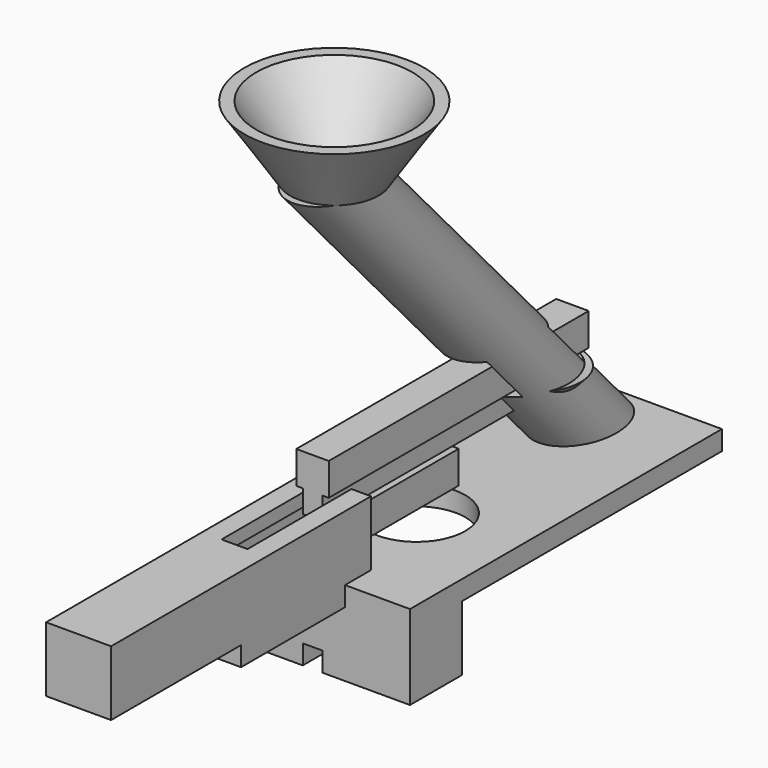
from build123d import *

# Parameters (mm, degrees)
F0_W          = 10
F0_H          = 10
F0_W_2        = 6
F0_H_2        = 6
F1_DEPTH      = 50
F2_W          = 4
F2_H          = 20
F3_DEPTH      = 3
F4_W          = 5
F4_H          = 5
F5_DEPTH      = 20
F7_DEPTH      = 25
F7_DEPTH_BACK = 25
F8_W          = 30
F8_H          = 80
F9_DEPTH      = 3
F10_R         = 7.5
F11_DEPTH     = 3.001
F12_W         = 30
F12_H         = 10
F13_DEPTH     = 10
F14_W         = 3
F14_H         = 10
F15_DEPTH     = 3
F16_R         = 1
F17_DEPTH     = 5
F18_W         = 6
F18_H         = 6
F19_DEPTH     = 2
F20_W         = 10
F20_H         = 20
F21_DEPTH     = 25
F25_W         = 7.5
F25_H         = 7.5
F26_DEPTH     = 33.5
F27_W         = 3
F27_H         = 3.5
F28_DEPTH     = 11.6
F29_W         = 34.4351846725
F29_H         = 17.5250470638
F30_DEPTH     = 605
F33_W         = 16.5032114089
F33_H         = 5.4589001536
F34_DEPTH     = 25


with BuildPart() as f1:
    # F0 (on Front) → F1 (new body)
    with BuildSketch(Plane.XZ):
        Rectangle(F0_W, F0_H)
        Rectangle(F0_W_2, F0_H_2, mode=Mode.SUBTRACT)
    extrude(amount=F1_DEPTH)

    # F2 (on face) → F3 (cut)
    with BuildSketch(Plane.XY.offset(5)):
        with Locations((0, -10)):
            Rectangle(F2_W, F2_H)
    extrude(amount=-F3_DEPTH, mode=Mode.SUBTRACT)

    # F8 (on face) → F9 (join)
    with BuildSketch(Plane(origin=(0, 0, -5), x_dir=(1, 0, 0), z_dir=(0, 0, -1))):
        with Locations((0, -15)):
            Rectangle(F8_W, F8_H)
    extrude(amount=F9_DEPTH)

    # F10 (on face) → F11 (cut, through all)
    with BuildSketch(Plane.XY.offset(-5)):
        with Locations((0, 15)):
            Circle(F10_R)
    extrude(amount=-F11_DEPTH, mode=Mode.SUBTRACT)

    # F12 (on face) → F13 (join)
    with BuildSketch(Plane(origin=(0, 0, -8), x_dir=(1, 0, 0), z_dir=(0, 0, -1))):
        Rectangle(F12_W, F12_H)
    extrude(amount=F13_DEPTH)

    # F14 (on face) → F15 (cut)
    with BuildSketch(Plane(origin=(0, 0, -18), x_dir=(1, 0, 0), z_dir=(0, 0, -1))):
        Rectangle(F14_W, F14_H)
    extrude(amount=-F15_DEPTH, mode=Mode.SUBTRACT)

    # F16 (on face) → F17 (cut)
    with BuildSketch(Plane(origin=(0, 0, -18), x_dir=(1, 0, 0), z_dir=(0, 0, -1))):
        with Locations((-5, 0)):
            Circle(F16_R)
        with Locations((5, 0)):
            Circle(F16_R)
    extrude(amount=-F17_DEPTH, mode=Mode.SUBTRACT)

    # F18 (on face) → F19 (join)
    with BuildSketch(Plane.XZ.offset(50)):
        Rectangle(F18_W, F18_H)
    extrude(amount=-F19_DEPTH)

    # F20 (on face) → F21 (cut)
    with BuildSketch(Plane.XY.offset(-5)):
        with Locations((-10, -15)):
            Rectangle(F20_W, F20_H)
        with Locations((10, -15)):
            Rectangle(F20_W, F20_H)
    extrude(amount=-F21_DEPTH, mode=Mode.SUBTRACT)

    # F22 (on Right) → F23 (revolve)
    with BuildSketch(Plane.YZ):
        Polygon((-2.0557420257, 53.4116236296), (52.0781588757, -5.8047241393), (54.0045872331, -4.9478402361), (-0.5796004863, 54.7610702405), align=None)
    revolve(axis=Axis((0, 22.938336782, 20.5131024087), (0, -0.6747233055, 0.7380707697)))

    # F25 (on offset) → F26 (cut)
    with BuildSketch(Plane(origin=(0, 55, 0), x_dir=(-1, 0, 0), z_dir=(0, 1, 0))):
        with Locations((-0.0233930768, 9.3513107755)):
            Rectangle(F25_W, F25_H)
    extrude(amount=-F26_DEPTH, mode=Mode.SUBTRACT)

    # F29 (on Right) → F30 (cut, symmetric)
    with BuildSketch(Plane.YZ):
        with Locations((-0.082434155, 55.3970336914)):
            Rectangle(F29_W, F29_H)
    extrude(amount=F30_DEPTH, both=True, mode=Mode.SUBTRACT)

    # F31 (on Right) → F32 (revolve)
    with BuildSketch(Plane.YZ):
        Polygon((11.19965408, 57.2443678975), (4.3785599992, 46.4661866426), (6.0238954611, 46.6490015388), (13.0396680906, 57.2443678975), align=None)
    revolve(axis=Axis((0, -0.8046502189, 52.2255096585), (0, 0, 1)))

    # F33 (on face) → F34 (cut)
    with BuildSketch(Plane.YZ.offset(15)):
        with Locations((46.7483942956, -10.7294500768)):
            Rectangle(F33_W, F33_H)
    extrude(amount=-F34_DEPTH, mode=Mode.SUBTRACT)

    # F35 (on Right) → F36 (revolve)
    with BuildSketch(Plane.YZ):
        Polygon((31.2420167029, 5.5713723414), (35.6345362961, 0.7823074702), (38.0581617355, 0.7823074702), (38.0581617355, 4.5863807123), align=None)
    revolve(axis=Axis((0, 38.0581617355, 2.6843440912), (0, 0, -1)))


with BuildPart() as f5:
    # F4 (on face) → F5 (new body)
    with BuildSketch(Plane(origin=(0, 0, 0), x_dir=(-1, 0, 0), z_dir=(0, 1, 0))):
        Rectangle(F4_W, F4_H)
    extrude(amount=F5_DEPTH)

    # F6 (on face) → F7 (join, two sides)
    with BuildSketch(Plane(origin=(0, 20, 0), x_dir=(-1, 0, 0), z_dir=(0, 1, 0))) as f7_sk:
        Polygon((-2.5, 11), (-2.5, 6), (-1.5, 6), (-1.5, 2.5), (1.5, 2.5), (1.5, 6), (2.5, 6), (2.5, 11), align=None)
    extrude(amount=F7_DEPTH)
    extrude(f7_sk.sketch, amount=-F7_DEPTH_BACK)

    # F27 (on face) → F28 (cut)
    with BuildSketch(Plane(origin=(0, 45, 0), x_dir=(-1, 0, 0), z_dir=(0, 1, 0))):
        with Locations((0, 4.25)):
            Rectangle(F27_W, F27_H)
    extrude(amount=-F28_DEPTH, mode=Mode.SUBTRACT)


solid = Compound([f1.part, f5.part])
